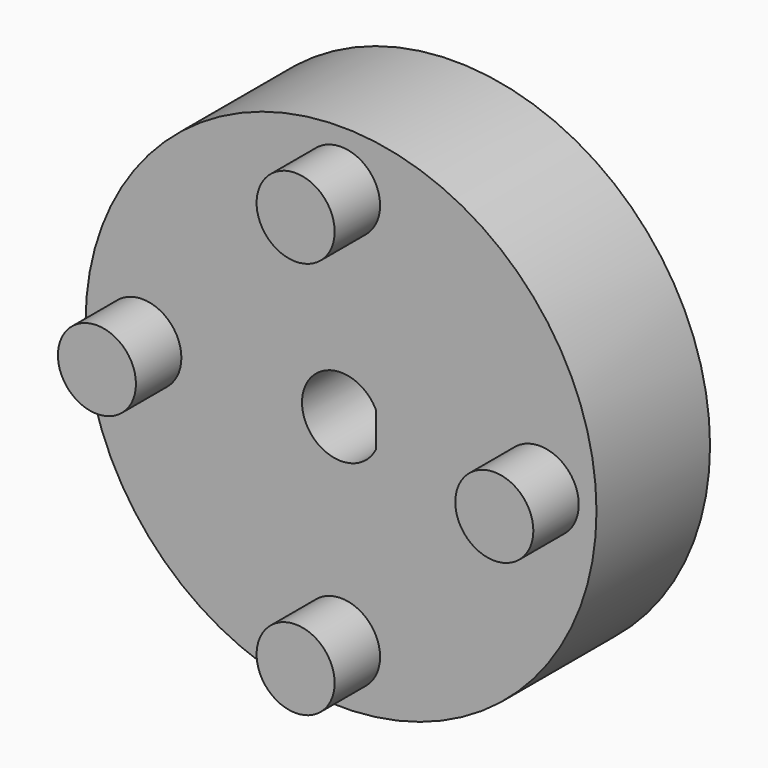
from build123d import *

# Parameters (mm, degrees)
F0_R     = 9
F0_R_2   = 1.375
F0_R_3   = 4
F1_DEPTH = 2
F2_DEPTH = 4
F3_DEPTH = 3


with BuildPart() as f1:
    # F0 (on Front) → F1 (new body)
    with BuildSketch(Plane.XZ):
        Circle(F0_R)
        with Locations((0, -7)):
            Circle(F0_R_2, mode=Mode.SUBTRACT)
        with Locations((-7, 0)):
            Circle(F0_R_2, mode=Mode.SUBTRACT)
        Circle(F0_R_3, mode=Mode.SUBTRACT)
        with Locations((7, 0)):
            Circle(F0_R_2, mode=Mode.SUBTRACT)
        with Locations((0, 7)):
            Circle(F0_R_2, mode=Mode.SUBTRACT)
        Circle(F0_R_3)
        with BuildLine():
            ThreePointArc((1.2252600864, 0.6239893595), (1.337041065, 0.3208522879), (1.375, 0))
            ThreePointArc((1.375, 0), (1.337041065, -0.3208522879), (1.2252600864, -0.6239893595))
            ThreePointArc((1.2252600864, -0.6239893595), (-1.375, 0), (1.2252600864, 0.6239893595))
        make_face(mode=Mode.SUBTRACT)
        with Locations((0, 7)):
            Circle(F0_R_2)
        with BuildLine():
            ThreePointArc((1.2252600864, -0.6239893595), (1.337041065, -0.3208522879), (1.375, 0))
            ThreePointArc((1.375, 0), (1.337041065, 0.3208522879), (1.2252600864, 0.6239893595))
            Line((1.2252600864, 0.6239893595), (1.2252600864, -0.6239893595))
        make_face()
    extrude(amount=F1_DEPTH)

    # F0 (on Front) → F2 (join)
    with BuildSketch(Plane.XZ):
        with Locations((-7, 0)):
            Circle(F0_R_2)
        with Locations((0, 7)):
            Circle(F0_R_2)
        with Locations((7, 0)):
            Circle(F0_R_2)
        with Locations((0, -7)):
            Circle(F0_R_2)
    extrude(amount=F2_DEPTH)

    # F0 (on Front) → F3 (join)
    with BuildSketch(Plane.XZ):
        Circle(F0_R)
        with Locations((0, -7)):
            Circle(F0_R_2, mode=Mode.SUBTRACT)
        with Locations((-7, 0)):
            Circle(F0_R_2, mode=Mode.SUBTRACT)
        Circle(F0_R_3, mode=Mode.SUBTRACT)
        with Locations((7, 0)):
            Circle(F0_R_2, mode=Mode.SUBTRACT)
        with Locations((0, 7)):
            Circle(F0_R_2, mode=Mode.SUBTRACT)
        Circle(F0_R_3)
        with BuildLine():
            ThreePointArc((1.2252600864, 0.6239893595), (1.337041065, 0.3208522879), (1.375, 0))
            ThreePointArc((1.375, 0), (1.337041065, -0.3208522879), (1.2252600864, -0.6239893595))
            ThreePointArc((1.2252600864, -0.6239893595), (-1.375, 0), (1.2252600864, 0.6239893595))
        make_face(mode=Mode.SUBTRACT)
        with Locations((7, 0)):
            Circle(F0_R_2)
        with Locations((0, 7)):
            Circle(F0_R_2)
        with Locations((-7, 0)):
            Circle(F0_R_2)
        with Locations((0, -7)):
            Circle(F0_R_2)
        with BuildLine():
            ThreePointArc((1.2252600864, -0.6239893595), (1.337041065, -0.3208522879), (1.375, 0))
            ThreePointArc((1.375, 0), (1.337041065, 0.3208522879), (1.2252600864, 0.6239893595))
            Line((1.2252600864, 0.6239893595), (1.2252600864, -0.6239893595))
        make_face()
    extrude(amount=-F3_DEPTH)


solid = f1.part
